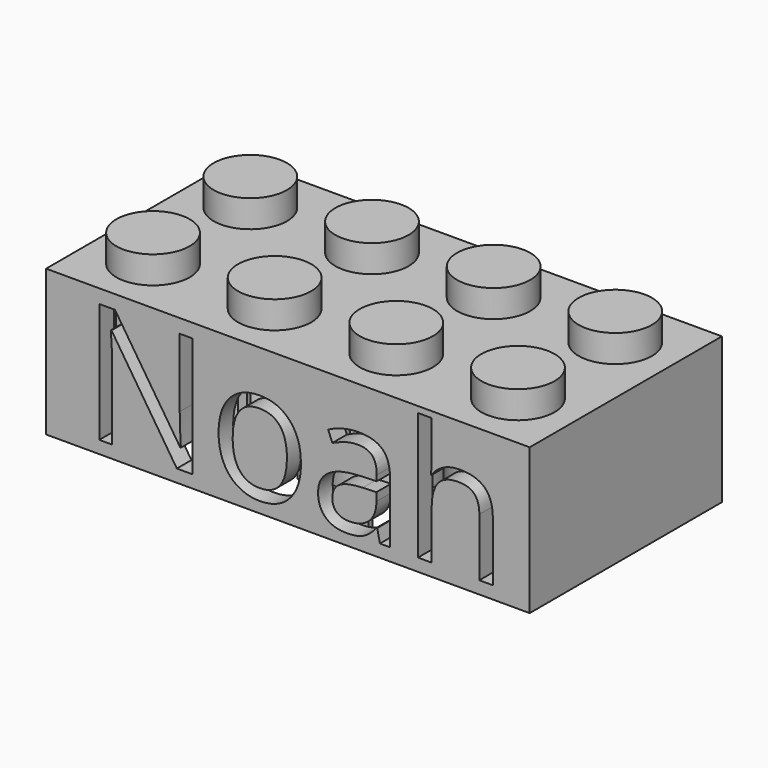
from build123d import *

# Parameters (mm, degrees)
F0_W          = 31.8
F0_H          = 15.8
F1_DEPTH      = 9.6
F2_W          = 29.4
F2_H          = 13.4
F3_DEPTH      = 8.4
F4_R          = 2.4089990553
F5_DEPTH      = 1.8
F6_R          = 1.3
F7_DEPTH      = 1.2
F8_R          = 3.255
F8_R_2        = 2.4
F9_DEPTH      = 8.4
F10_W         = 0.6
F10_H         = 0.3
F11_DEPTH     = 8.4
F12_W         = 0.3
F12_H         = 0.6
F13_DEPTH     = 8.4
F15_TEXT_SIZE = 11.0174210729
F16_DEPTH     = 1.2
F14_W         = 0.6594991025
F14_H         = 4.3966606837
F14_W_2       = 0.6
F14_H_2       = 4
F17_DEPTH     = 6.4


# Not quite as in the source:
# - Text() gives the source's letters only with a copy of the font that has no kerning and outlines rounded to 1/6400 em; it was checked with that copy


with BuildPart() as f1:
    # F0 (on Top) → F1 (new body)
    with BuildSketch(Plane.XY):
        Rectangle(F0_W, F0_H)
    extrude(amount=F1_DEPTH)

    # F2 (on Top) → F3 (cut)
    with BuildSketch(Plane.XY):
        Rectangle(F2_W, F2_H)
    extrude(amount=F3_DEPTH, mode=Mode.SUBTRACT)

    # F4 (on face) → F5 (join)
    with BuildSketch(Plane.XY.offset(9.6)):
        with Locations((-11.95, 3.95)):
            Circle(F4_R)
        with Locations((-11.95, -4.05)):
            Circle(F4_R)
        with Locations((-3.95, 3.95)):
            Circle(F4_R)
        with Locations((-3.95, -4.05)):
            Circle(F4_R)
        with Locations((4.05, 3.95)):
            Circle(F4_R)
        with Locations((4.05, -4.05)):
            Circle(F4_R)
        with Locations((12.05, 3.95)):
            Circle(F4_R)
        with Locations((12.05, -4.05)):
            Circle(F4_R)
    extrude(amount=F5_DEPTH)

    # F6 (on face) → F7 (cut)
    with BuildSketch(Plane(origin=(0, 0, 8.4), x_dir=(1, 0, 0), z_dir=(0, 0, -1))):
        with Locations((-11.95, 3.95)):
            Circle(F6_R)
        with Locations((-11.95, -4.05)):
            Circle(F6_R)
        with Locations((-3.95, 3.95)):
            Circle(F6_R)
        with Locations((-3.95, -4.05)):
            Circle(F6_R)
        with Locations((4.05, 3.95)):
            Circle(F6_R)
        with Locations((4.05, -4.05)):
            Circle(F6_R)
        with Locations((12.05, 3.95)):
            Circle(F6_R)
        with Locations((12.05, -4.05)):
            Circle(F6_R)
    extrude(amount=-F7_DEPTH, mode=Mode.SUBTRACT)

    # F8 (on face) → F9 (join, through all)
    with BuildSketch(Plane(origin=(0, 0, 8.4), x_dir=(1, 0, 0), z_dir=(0, 0, -1))):
        with Locations((-7.95, -0.05)):
            Circle(F8_R)
        with Locations((-7.95, -0.05)):
            Circle(F8_R_2, mode=Mode.SUBTRACT)
        with Locations((0.05, -0.05)):
            Circle(F8_R)
        with Locations((0.05, -0.05)):
            Circle(F8_R_2, mode=Mode.SUBTRACT)
        with Locations((8.05, -0.05)):
            Circle(F8_R)
        with Locations((8.05, -0.05)):
            Circle(F8_R_2, mode=Mode.SUBTRACT)
    extrude(amount=F9_DEPTH)

    # F10 (on face) → F11 (join, through all)
    with BuildSketch(Plane(origin=(0, 0, 0), x_dir=(1, 0, 0), z_dir=(0, 0, -1))):
        with Locations((-11.95, 6.55)):
            Rectangle(F10_W, F10_H)
        with Locations((-11.95, -6.55)):
            Rectangle(F10_W, F10_H)
        with Locations((-3.95, 6.55)):
            Rectangle(F10_W, F10_H)
        with Locations((-3.95, -6.55)):
            Rectangle(F10_W, F10_H)
        with Locations((4.05, 6.55)):
            Rectangle(F10_W, F10_H)
        with Locations((4.05, -6.55)):
            Rectangle(F10_W, F10_H)
        with Locations((12.05, 6.55)):
            Rectangle(F10_W, F10_H)
        with Locations((12.05, -6.55)):
            Rectangle(F10_W, F10_H)
    extrude(amount=-F11_DEPTH)

    # F12 (on face) → F13 (join, through all)
    with BuildSketch(Plane(origin=(0, 0, 0), x_dir=(1, 0, 0), z_dir=(0, 0, -1))):
        with Locations((-14.55, 3.95)):
            Rectangle(F12_W, F12_H)
        with Locations((-14.55, -4.05)):
            Rectangle(F12_W, F12_H)
        with Locations((14.55, 3.95)):
            Rectangle(F12_W, F12_H)
        with Locations((14.55, -4.05)):
            Rectangle(F12_W, F12_H)
    extrude(amount=-F13_DEPTH)

    # F15 (on face) → F16 (cut)
    with BuildSketch(Plane.XZ.offset(7.9)):
        with Locations((-13.481708302, 0.8260054747)):
            Text('Noah', F15_TEXT_SIZE, font='Open Sans', text_align=(TextAlign.LEFT, TextAlign.BOTTOM))
    extrude(amount=-F16_DEPTH, mode=Mode.SUBTRACT)

    # F14 (on face) → F17 (join)
    with BuildSketch(Plane(origin=(0, 0, 8.4), x_dir=(1, 0, 0), z_dir=(0, 0, -1))):
        with Locations((-0.0049582585, 4.5016696582)):
            Rectangle(F14_W, F14_H)
        with Locations((0, -4.7)):
            Rectangle(F14_W_2, F14_H_2)
    extrude(amount=F17_DEPTH)


solid = f1.part
